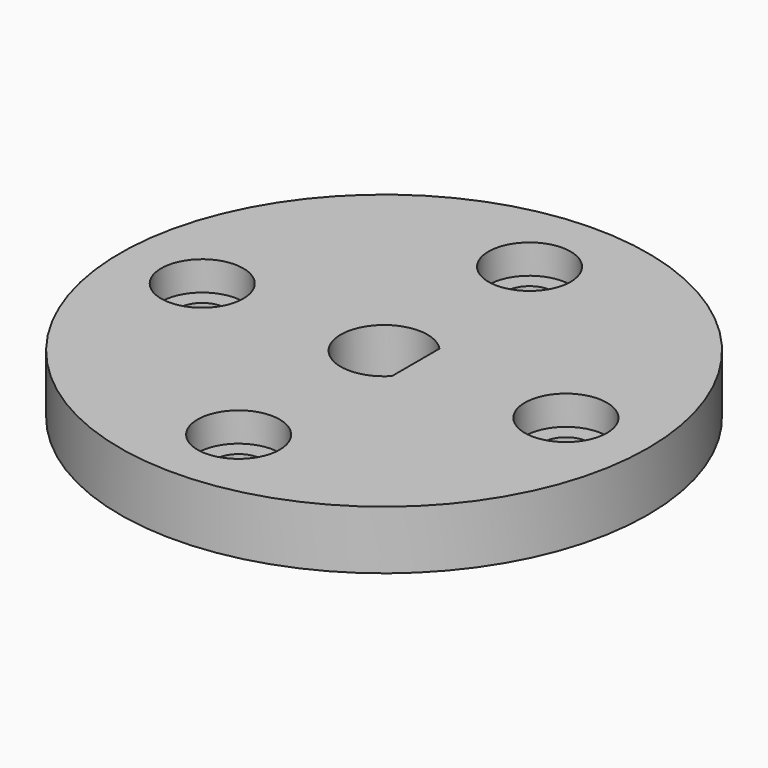
from build123d import *

# Parameters (mm, degrees)
F0_R     = 22.5
F1_DEPTH = 5
F3_DEPTH = 25
F5_DEPTH = 25
F6_R     = 2
F7_DEPTH = 25
F8_R     = 3.5
F9_DEPTH = 2.5


with BuildPart() as f1:
    # F0 (on Top) → F1 (new body)
    with BuildSketch(Plane.XY):
        Circle(F0_R)
    extrude(amount=F1_DEPTH)

    # F2 (on face) → F3 (cut)
    with BuildSketch(Plane.XY.offset(5)):
        with BuildLine():
            Line((2.7, 0), (2.7, 2.5298221281))
            ThreePointArc((2.7, 2.5298221281), (-3.7, 0), (2.7, -2.5298221281))
            Line((2.7, -2.5298221281), (2.7, 0))
        make_face()
    extrude(amount=-F3_DEPTH, mode=Mode.SUBTRACT)

    # F4 (on face) → F5 (cut)
    with BuildSketch(Plane.XY.offset(5)):
        with BuildLine():
            ThreePointArc((0, 17.5), (-1.4142135624, 14.0857864376), (2, 15.5))
            ThreePointArc((2, 15.5), (1.4142135624, 16.9142135624), (0, 17.5))
        make_face()
    extrude(amount=-F5_DEPTH, mode=Mode.SUBTRACT)

    # F6 (on face) → F7 (cut)
    with BuildSketch(Plane.XY.offset(5)):
        with Locations((15.5, 0)):
            Circle(F6_R)
        with BuildLine():
            ThreePointArc((0, -17.5), (1.4142135624, -16.9142135624), (2, -15.5))
            ThreePointArc((2, -15.5), (-1.4142135624, -14.0857864376), (0, -17.5))
        make_face()
        with BuildLine():
            ThreePointArc((-17.5, 0), (-15.5, -2), (-13.5, 0))
            ThreePointArc((-13.5, 0), (-15.5, 2), (-17.5, 0))
        make_face()
    extrude(amount=-F7_DEPTH, mode=Mode.SUBTRACT)

    # F8 (on face) → F9 (cut)
    with BuildSketch(Plane.XY.offset(5)):
        with Locations((-15.5, 0)):
            Circle(F8_R)
        with Locations((15.5, 0)):
            Circle(F8_R)
        with Locations((0, -15.5)):
            Circle(F8_R)
        with Locations((0, 15.5)):
            Circle(F8_R)
    extrude(amount=-F9_DEPTH, mode=Mode.SUBTRACT)


solid = f1.part
